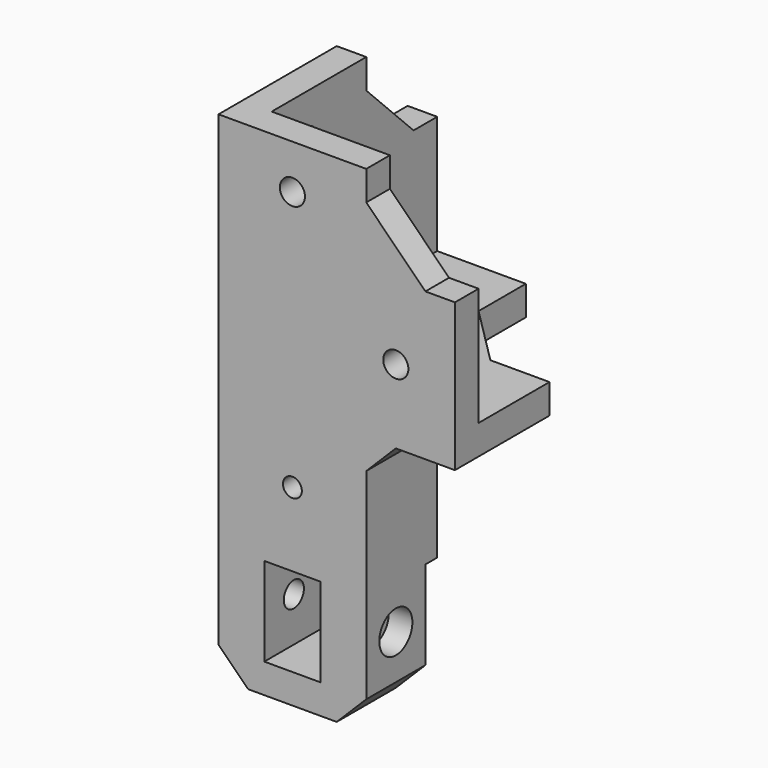
from build123d import *

# Parameters (mm, degrees)
F0_R         = 2.125
F1_DEPTH     = 5
F3_DEPTH     = 20
F5_DEPTH     = 15
F6_SIZE      = 10
F7_R         = 2.125
F8_DEPTH     = 5
F9_R         = 2.125
F10_DEPTH    = 5
F11_W        = 40
F11_H        = 20
F11_R        = 2.125
F12_DEPTH    = 24
F13_R        = 4.25
F14_DEPTH    = 25
F15_R        = 3.5
F16_DEPTH    = 25
F17_R        = 4.25
F17_R_2      = 1.6
F18_DEPTH    = 5
F19_T4_DEPTH = 20
F19_S5_R     = 2.125
F19_T6_DEPTH = 12
F19_T7_DEPTH = 36.8584149398
F21_DEPTH    = 12.5
F22_SIZE     = 5
F23_R        = 3.5
F24_DEPTH    = 44.001
F25_R        = 2.125
F26_DEPTH    = 40.001
F28_DEPTH    = 4
F29_R        = 3.5
F30_DEPTH    = 4


# Not quite as in the source:
# - a fillet or chamfer that OpenCascade refuses, or shapes differently, is made with other operations: its cross-section is extruded or revolved along the edge and cut away or added


with BuildPart() as f1:
    # F0 (on Top) → F1 (new body)
    with BuildSketch(Plane.XY):
        Polygon((0, 20), (0, 40), (-20, 40), (-20, 0), (20, 0), (20, 20), align=None)
        with Locations((-7.5, 12.5)):
            Circle(F0_R, mode=Mode.SUBTRACT)
        with Locations((10, 12.5)):
            Circle(F0_R, mode=Mode.SUBTRACT)
        with Locations((-7.5, 30)):
            Circle(F0_R, mode=Mode.SUBTRACT)
    extrude(amount=F1_DEPTH)

    # F2 (on face) → F3 (join)
    with BuildSketch(Plane.XY.offset(5)):
        Polygon((-15, 40), (-20, 40), (-20, 0), (20, 0), (20, 5), (-15, 5), align=None)
    extrude(amount=F3_DEPTH)

    # F4 (on face) → F5 (join)
    with BuildSketch(Plane.XY.offset(25)):
        Polygon((-15, 5), (-15, 25), (-20, 25), (-20, 0), (5, 0), (5, 5), align=None)
    extrude(amount=F5_DEPTH)

    # F6
    f6_edges = [f1.edges().sort_by_distance(p)[0] for p in [
        (0, 20, 2.5),
        (-17.5, 25, 25),
        (5, 2.5, 25),
    ]]
    chamfer(f6_edges, length=F6_SIZE)

    # F7 (on face) → F8 (cut)
    with BuildSketch(Plane.XZ):
        with Locations((-7.5, 32.5)):
            Circle(F7_R)
        with Locations((10, 12.5)):
            Circle(F7_R)
    extrude(amount=-F8_DEPTH, mode=Mode.SUBTRACT)

    # F9 (on face) → F10 (cut)
    with BuildSketch(Plane(origin=(-20, 0, 0), x_dir=(0, -1, 0), z_dir=(-1, 0, 0))):
        with Locations((-12.5, 32.5)):
            Circle(F9_R)
        with Locations((-30, 12.5)):
            Circle(F9_R)
    extrude(amount=-F10_DEPTH, mode=Mode.SUBTRACT)

    # F11 (on face) → F12 (join)
    with BuildSketch(Plane(origin=(0, 0, 0), x_dir=(1, 0, 0), z_dir=(0, 0, -1))):
        with Locations((0, -10)):
            Rectangle(F11_W, F11_H)
        with Locations((-7.5, -12.5)):
            Circle(F11_R, mode=Mode.SUBTRACT)
        with Locations((10, -12.5)):
            Circle(F11_R, mode=Mode.SUBTRACT)
    extrude(amount=F12_DEPTH)

    # F13 (on face) → F14 (cut)
    with BuildSketch(Plane(origin=(0, 20, 0), x_dir=(-1, 0, 0), z_dir=(0, 1, 0))):
        with Locations((7.5, -11.5)):
            Circle(F13_R)
        Polygon((-5, -24), (-5, -11.5), (-5, 0), (-20, 0), (-20, -24), align=None)
    extrude(amount=-F14_DEPTH, mode=Mode.SUBTRACT)

    # F15 (on face) → F16 (cut)
    with BuildSketch(Plane(origin=(0, 0, 0), x_dir=(1, 0, 0), z_dir=(0, 0, -1))):
        with Locations((-7.5, -12.5)):
            Circle(F15_R)
    extrude(amount=F16_DEPTH, mode=Mode.SUBTRACT)

    # F17 (on face) → F18 (join)
    with BuildSketch(Plane.XZ):
        with Locations((-7.5, -11.5)):
            Circle(F17_R)
        with Locations((-7.5, -11.5)):
            Circle(F17_R_2, mode=Mode.SUBTRACT)
    extrude(amount=-F18_DEPTH)

    # F19: chamfer of 5 on 2 edges, made by hand


with BuildPart() as f19_tool2:
    # F19_s3 → F19_t4 (new body)
    with BuildSketch(Plane.XZ.offset(-20)):
        Polygon((5, -5), (10, 0), (5, 0), align=None)
    extrude(amount=F19_T4_DEPTH)

    # F19_s5 → F19_t6 (cut, symmetric)
    with BuildSketch(Plane.XY.offset(-2.5)):
        with Locations((10, 12.5)):
            Circle(F19_S5_R)
    extrude(amount=F19_T6_DEPTH, both=True, mode=Mode.SUBTRACT)


with BuildPart() as f1_1:
    add(f1.part)

    # F19_t1: union F19_tool2
    add(f19_tool2.part)

    # F19_s8 → F19_t7 (cut)
    with BuildSketch(Plane.XY.offset(-36.8584149398)):
        Polygon((-20, 15), (-15, 20), (-20, 20), align=None)
    extrude(amount=F19_T7_DEPTH, mode=Mode.SUBTRACT)

    # F20 (on face) → F21 (join)
    with BuildSketch(Plane.XZ):
        Polygon((-12.25, -24), (-20, -24), (-20, -44), (5, -44), (5, -24), (-2.75, -24), (-2.75, -39), (-12.25, -39), align=None)
    extrude(amount=-F21_DEPTH)

    # F22
    f22_edges = [f1_1.edges().sort_by_distance(p)[0] for p in [
        (-20, 6.25, -44),
        (5, 6.25, -44),
        (5, 20, -14.5),
    ]]
    chamfer(f22_edges, length=F22_SIZE)

    # F23 (on face) → F24 (cut, through all)
    with BuildSketch(Plane(origin=(0, 0, 0), x_dir=(1, 0, 0), z_dir=(0, 0, -1))):
        with Locations((10, -12.5)):
            Circle(F23_R)
    extrude(amount=F24_DEPTH, mode=Mode.SUBTRACT)

    # F25 (on face) → F26 (cut, through all)
    with BuildSketch(Plane(origin=(-20, 0, 0), x_dir=(0, -1, 0), z_dir=(-1, 0, 0))):
        with Locations((-6.25, -31.5)):
            Circle(F25_R)
    extrude(amount=-F26_DEPTH, mode=Mode.SUBTRACT)

    # F27 (on face) → F28 (cut)
    with BuildSketch(Plane(origin=(-20, 0, 0), x_dir=(0, -1, 0), z_dir=(-1, 0, 0))):
        Polygon((-3.325, -33.1887495374), (-3.325, -29.8112504626), (-6.25, -28.1225009252), (-9.175, -29.8112504626), (-9.175, -33.1887495374), (-6.25, -34.8774990748), align=None)
    extrude(amount=-F28_DEPTH, mode=Mode.SUBTRACT)

    # F29 (on face) → F30 (cut)
    with BuildSketch(Plane.YZ.offset(5)):
        with Locations((6.25, -31.5)):
            Circle(F29_R)
    extrude(amount=-F30_DEPTH, mode=Mode.SUBTRACT)


solid = f1_1.part
